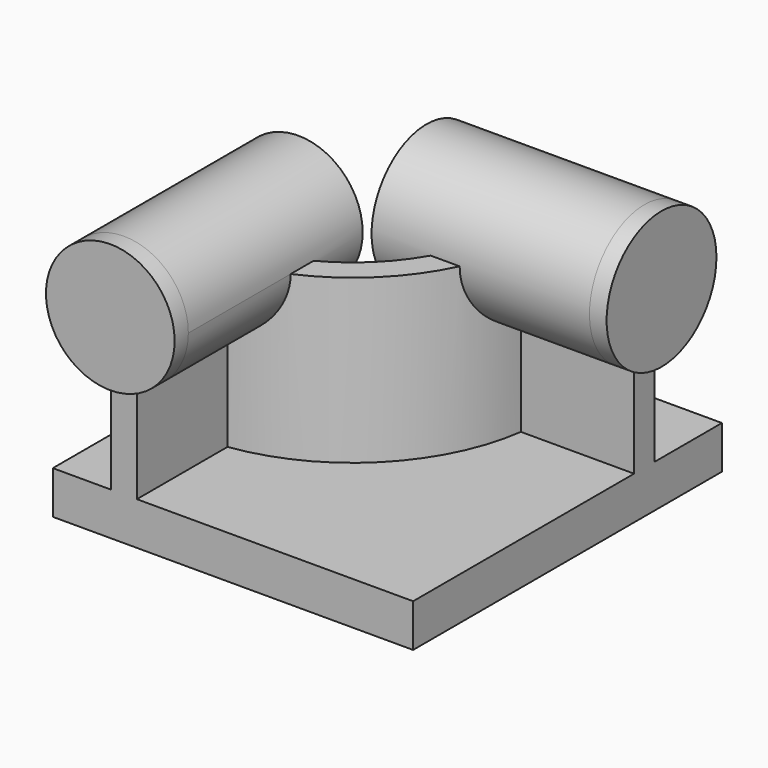
from build123d import *

# Parameters (mm, degrees)
F0_W          = 210
F0_H          = 225
F1_DEPTH      = 25
F3_DEPTH      = 95
F4_R          = 40
F5_DEPTH      = 10
F5_DEPTH_BACK = 127
F6_R          = 37.5
F7_DEPTH      = 10
F7_DEPTH_BACK = 127


with BuildPart() as f1:
    # F0 (on Top) → F1 (new body)
    with BuildSketch(Plane.XY):
        Rectangle(F0_W, F0_H)
    extrude(amount=F1_DEPTH)

    # F2 (on face) → F3 (join)
    with BuildSketch(Plane.XY.offset(25)):
        with BuildLine():
            Line((-71, -32.5), (-71, -112.5))
            Line((-71, -112.5), (-56, -112.5))
            Line((-56, -112.5), (-56, -46.4818166789))
            ThreePointArc((-56, -46.4818166789), (7.4888527117, -14.9888527117), (38.9818166789, 48.5))
            Line((38.9818166789, 48.5), (105, 48.5))
            Line((105, 48.5), (105, 63.5))
            Line((105, 63.5), (25, 63.5))
            ThreePointArc((25, 63.5), (-3.1177490061, -4.3822509939), (-71, -32.5))
        make_face()
    extrude(amount=F3_DEPTH)

    # F4 (on face) → F5 (join, two sides)
    with BuildSketch(Plane.YZ.offset(105)) as f5_sk:
        with Locations((56, 120)):
            Circle(F4_R)
    extrude(amount=F5_DEPTH)
    extrude(f5_sk.sketch, amount=-F5_DEPTH_BACK)

    # F6 (on face) → F7 (join, two sides)
    with BuildSketch(Plane.XZ.offset(112.5)) as f7_sk:
        with Locations((-63.5, 120)):
            Circle(F6_R)
        with BuildLine():
            ThreePointArc((-56, 83.2576538583), (-34.4526249034, 96.2829175487), (-26, 120))
            ThreePointArc((-26, 120), (-87.2170824513, 149.0473750966), (-71, 83.2576538583))
            Line((-71, 83.2576538583), (-71, 120))
            Line((-71, 120), (-56, 120))
            Line((-56, 120), (-56, 83.2576538583))
        make_face()
    extrude(amount=F7_DEPTH)
    extrude(f7_sk.sketch, amount=-F7_DEPTH_BACK)


solid = f1.part
